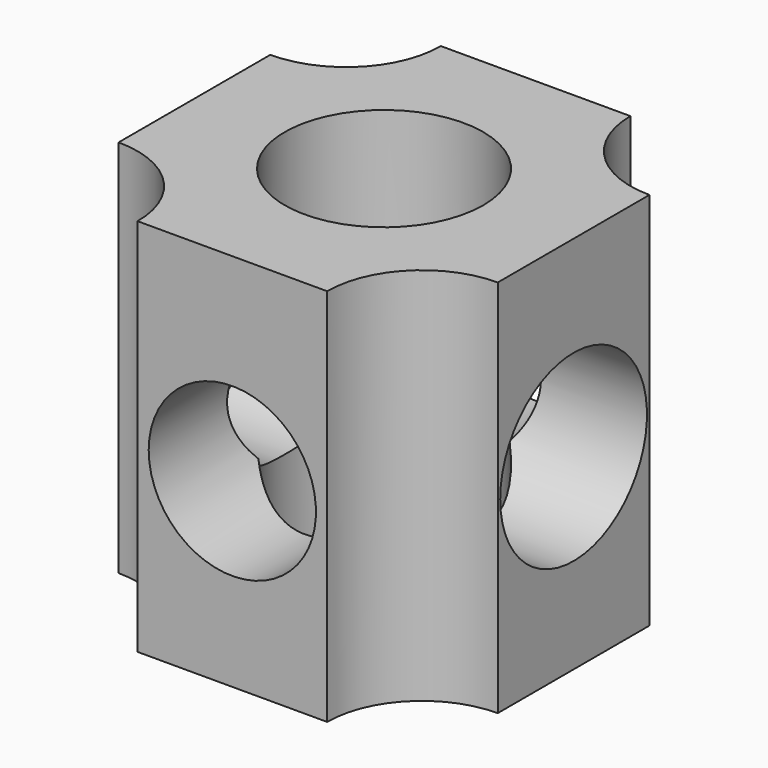
from build123d import *

# Parameters (mm, degrees)
F0_W      = 100
F0_H      = 100
F1_DEPTH  = 100
F2_R      = 26.1687098173
F3_DEPTH  = 100
F4_W      = 25
F4_H      = 25
F5_DEPTH  = 125.4000663757
F6_R      = 24.99999
F7_R      = 24.1891086676
F8_DEPTH  = 116.3376644254
F9_R      = 22.0548114827
F10_DEPTH = 146.7472165823


# Not quite as in the source:
# - a fillet or chamfer is up to 0.001 mm smaller than in the source, because OpenCascade refuses the exact size


with BuildPart() as f1:
    # F0 (on Top) → F1 (new body)
    with BuildSketch(Plane.XY):
        Rectangle(F0_W, F0_H)
    extrude(amount=F1_DEPTH)

    # F2 (on face) → F3 (cut)
    with BuildSketch(Plane.XY.offset(100)):
        Circle(F2_R)
    extrude(amount=-F3_DEPTH, mode=Mode.SUBTRACT)

    # F4 (on face) → F5 (cut)
    with BuildSketch(Plane.XY.offset(100)):
        with Locations((37.5, 37.5)):
            Rectangle(F4_W, F4_H)
        with Locations((-37.5, 37.5)):
            Rectangle(F4_W, F4_H)
        with Locations((-37.5, -37.5)):
            Rectangle(F4_W, F4_H)
        with Locations((37.5, -37.5)):
            Rectangle(F4_W, F4_H)
    extrude(amount=-F5_DEPTH, mode=Mode.SUBTRACT)

    # F6 (radius 25 in the source; OpenCascade refuses exactly that, so slightly less here)
    f6_edges = [f1.edges().sort_by_distance(p)[0] for p in [
        (-25, -25, 50),
        (25, -25, 50),
        (25, 25, 50),
        (-25, 25, 50),
    ]]
    fillet(f6_edges, radius=F6_R)

    # F7 (on face) → F8 (cut)
    with BuildSketch(Plane(origin=(-50, 0, 0), x_dir=(0, -1, 0), z_dir=(-1, 0, 0))):
        with Locations((0, 49.3326857686)):
            Circle(F7_R)
    extrude(amount=-F8_DEPTH, mode=Mode.SUBTRACT)

    # F9 (on face) → F10 (cut)
    with BuildSketch(Plane(origin=(0, 50, 0), x_dir=(-1, 0, 0), z_dir=(0, 1, 0))):
        with Locations((0, 47.8064343333)):
            Circle(F9_R)
    extrude(amount=-F10_DEPTH, mode=Mode.SUBTRACT)


solid = f1.part
